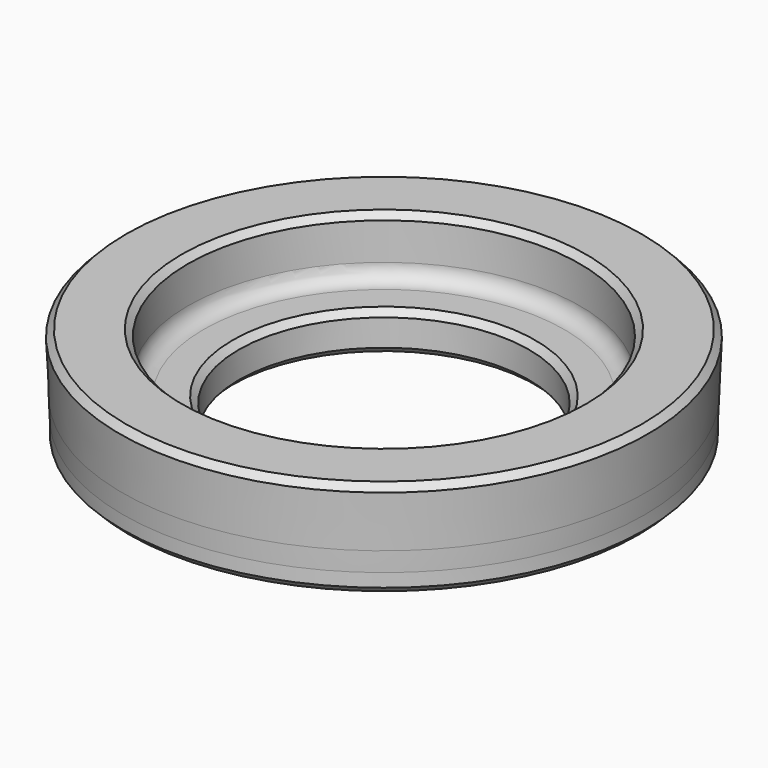
from build123d import *


# Not quite as in the source:
# - a fillet or chamfer that OpenCascade refuses, or shapes differently, is made with other operations: its cross-section is extruded or revolved along the edge and cut away or added


with BuildPart() as f1:
    # F0 (on Front) → F1 (revolve)
    with BuildSketch(Plane.XZ):
        with BuildLine():
            Line((-66.7483291848, 10), (-66.5397158787, 5))
            Line((-66.5397158787, 5), (-66.5397158787, 0))
            Line((-66.5397158787, 0), (-37, 0))
            Line((-37, 0), (-37, 10))
            Line((-37, 10), (-46, 10))
            ThreePointArc((-46, 10), (-48.8284271247, 11.1715728753), (-50, 14))
            Line((-50, 14), (-50, 25.0225278729))
            Line((-50, 25.0225278729), (-67.375109026, 25.0225278729))
            Line((-67.375109026, 25.0225278729), (-66.7483291848, 10))
        make_face()
    revolve(axis=Axis((0, 0, 30.7617206126), (0, 0, 1)))

    # F2: chamfer of 1.6 on 5 edges, made by hand

    # F2_s1 → F2_t2 (revolve, cut)
    with BuildSketch(Plane.XZ):
        Polygon((-38.6, 10), (-37, 8.4), (-37, 10), align=None)
    revolve(axis=Axis((0, 0, 10), (0, 0, 1)), mode=Mode.SUBTRACT)

    # F2_s3 → F2_t4 (revolve, cut)
    with BuildSketch(Plane.XZ):
        Polygon((-37, 1.6), (-38.6, 0), (-37, 0), align=None)
    revolve(axis=Axis((0, 0, 0), (0, 0, 1)), mode=Mode.SUBTRACT)

    # F2_s5 → F2_t6 (revolve, cut)
    with BuildSketch(Plane.XZ):
        Polygon((-64.9397158787, 0), (-66.5397158787, 1.6), (-66.5397158787, 0), align=None)
    revolve(axis=Axis((0, 0, 0), (0, 0, 1)), mode=Mode.SUBTRACT)

    # F2_s7 → F2_t8 (revolve, cut)
    with BuildSketch(Plane.XZ):
        Polygon((-51.6, 25.0225278729), (-50, 23.4225278729), (-50, 25.0225278729), align=None)
    revolve(axis=Axis((0, 0, 25.0225278729), (0, 0, 1)), mode=Mode.SUBTRACT)

    # F2_s9 → F2_t10 (revolve, cut)
    with BuildSketch(Plane.XZ):
        Polygon((-67.3055699404, 23.3558296431), (-65.7069607492, 25.0225278729), (-67.375109026, 25.0225278729), align=None)
    revolve(axis=Axis((0, 0, 25.0225278729), (0, 0, 1)), mode=Mode.SUBTRACT)


solid = f1.part
